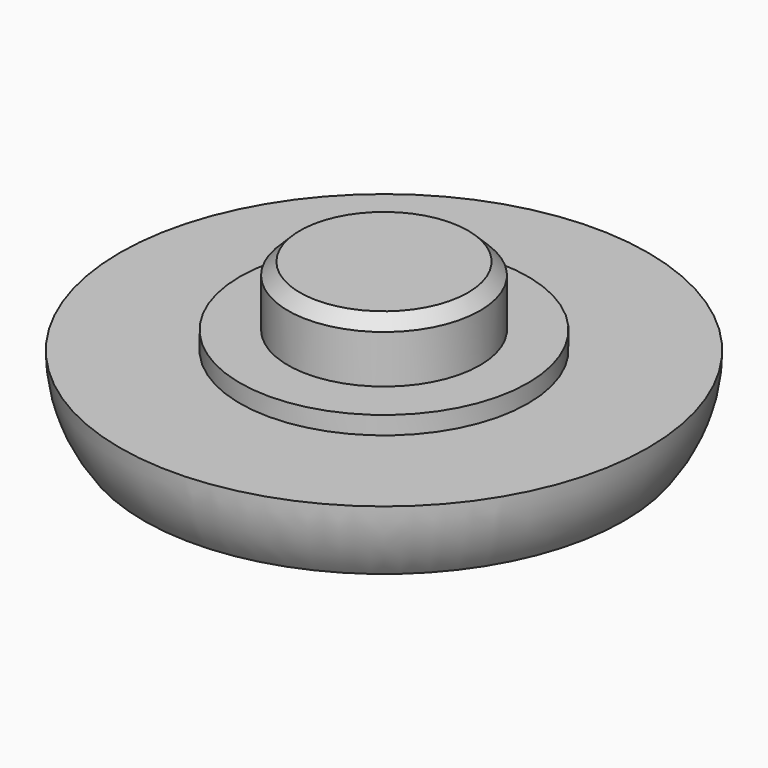
from build123d import *

# Parameters (mm, degrees)
F3_SIZE = 0.5


# Not quite as in the source:
# - a fillet or chamfer that OpenCascade refuses, or shapes differently, is made with other operations: its cross-section is extruded or revolved along the edge and cut away or added


with BuildPart() as f1:
    # F0 (on Front) → F1 (revolve)
    with BuildSketch(Plane.XZ):
        with BuildLine():
            Line((4, 6.25), (0, 6.25))
            Line((0, 6.25), (0, 0.75))
            add(Edge.make_bspline(
                [(10, 0), (10, 0.75), (0, 0.75)],
                knots=[0, 0, 0, 1.5707963268, 1.5707963268, 1.5707963268], degree=2, weights=[1, 0.7071067812, 1]))
            Line((10, 0), (11, 0))
            Line((11, 0), (11, 3))
            Line((11, 3), (6, 3))
            Line((6, 3), (6, 3.75))
            Line((6, 3.75), (4, 3.75))
            Line((4, 3.75), (4, 6.25))
        make_face()
    revolve(axis=Axis((0, 0, 3.5), (0, 0, -1)))

    # F2: fillet of radius 5 on 1 edges, made by hand

    # F2_s1 → F2_t2 (revolve, cut)
    with BuildSketch(Plane.XZ):
        with BuildLine():
            ThreePointArc((10, 0), (10.7434164903, 1.4188611699), (11, 3))
            Line((11, 3), (11, 0))
            Line((11, 0), (10, 0))
        make_face()
    revolve(axis=Axis((0, 0, 0), (0, 0, -1)), mode=Mode.SUBTRACT)

    # F3
    f3_edges = [f1.edges().sort_by_distance(p)[0] for p in [
        (-4, 0, 6.25),
    ]]
    chamfer(f3_edges, length=F3_SIZE)


solid = f1.part
